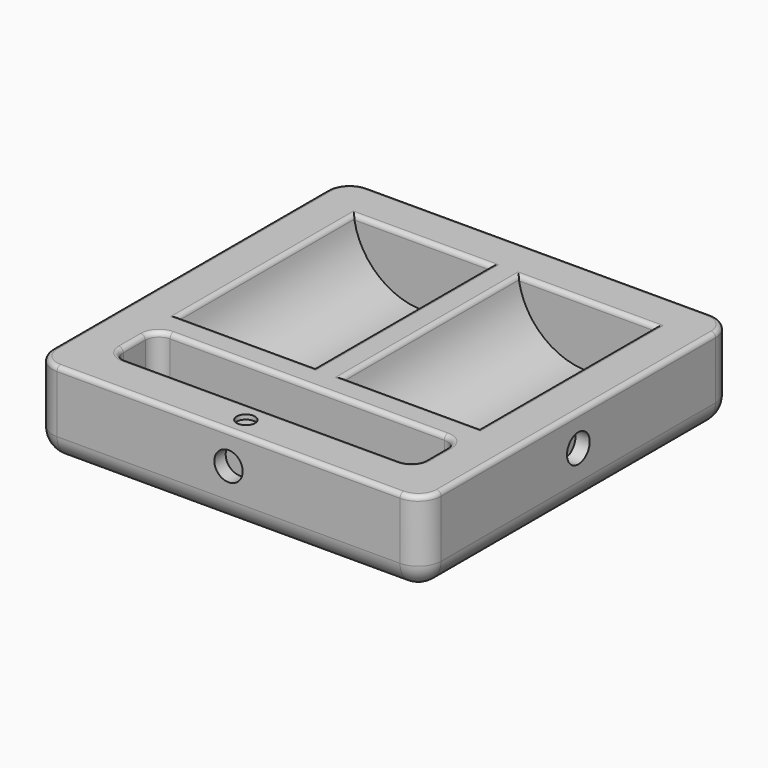
from build123d import *

# Parameters (mm, degrees)
F0_W      = 85
F0_H      = 85
F0_R      = 2
F3_DEPTH  = 18.5
F4_DEPTH  = 14
F5_R      = 5
F6_R      = 3
F7_R      = 3.1
F8_DEPTH  = 3.1
F9_R      = 3.1
F10_DEPTH = 3.1
F11_R     = 3.1
F12_DEPTH = 3.1
F13_R     = 3.1
F14_DEPTH = 3.1
F15_DEPTH = 1
F18_DEPTH = 48
F19_R     = 1
F20_ANGLE = 180


# Not quite as in the source:
# - a feature names something its author has since deleted; it is built from what else it names


with BuildPart() as f3:
    # F0 (on Top) → F3 (new body)
    with BuildSketch(Plane.XY):
        Rectangle(F0_W, F0_H)
        with BuildLine():
            ThreePointArc((-33, 30), (-32.1213203436, 32.1213203436), (-30, 33))
            Line((-30, 33), (30, 33))
            ThreePointArc((30, 33), (32.1213203436, 32.1213203436), (33, 30))
            Line((33, 30), (33, 24))
            ThreePointArc((33, 24), (32.1213203436, 21.8786796564), (30, 21))
            Line((30, 21), (-30, 21))
            ThreePointArc((-30, 21), (-32.1213203436, 21.8786796564), (-33, 24))
            Line((-33, 24), (-33, 30))
        make_face(mode=Mode.SUBTRACT)
        with Locations((0, 37.75)):
            Circle(F0_R, mode=Mode.SUBTRACT)
        with BuildLine():
            Line((30, 33), (-30, 33))
            ThreePointArc((-30, 33), (-32.1213203436, 32.1213203436), (-33, 30))
            Line((-33, 30), (-33, 24))
            ThreePointArc((-33, 24), (-32.1213203436, 21.8786796564), (-30, 21))
            Line((-30, 21), (30, 21))
            ThreePointArc((30, 21), (32.1213203436, 21.8786796564), (33, 24))
            Line((33, 24), (33, 30))
            ThreePointArc((33, 30), (32.1213203436, 32.1213203436), (30, 33))
        make_face()
        with Locations((0, 37.75)):
            Circle(F0_R)
    extrude(amount=F3_DEPTH)

    # F0 (on Top) → F4 (cut)
    with BuildSketch(Plane.XY):
        with BuildLine():
            Line((30, 33), (-30, 33))
            ThreePointArc((-30, 33), (-32.1213203436, 32.1213203436), (-33, 30))
            Line((-33, 30), (-33, 24))
            ThreePointArc((-33, 24), (-32.1213203436, 21.8786796564), (-30, 21))
            Line((-30, 21), (30, 21))
            ThreePointArc((30, 21), (32.1213203436, 21.8786796564), (33, 24))
            Line((33, 24), (33, 30))
            ThreePointArc((33, 30), (32.1213203436, 32.1213203436), (30, 33))
        make_face()
    extrude(amount=F4_DEPTH, mode=Mode.SUBTRACT)

    # F5
    f5_edges = [f3.edges().sort_by_distance(p)[0] for p in [
        (0, 42.5, 18.5),
        (-42.5, 0, 18.5),
        (0, -42.5, 18.5),
        (42.5, 0, 18.5),
        (42.5, 42.5, 9.25),
        (-42.5, 42.5, 9.25),
        (-42.5, -42.5, 9.25),
        (42.5, -42.5, 9.25),
    ]]
    fillet(f5_edges, radius=F5_R)

    # F6
    f6_edges = [f3.edges().sort_by_distance(p)[0] for p in [
        (0, 33, 14),
        (-32.12132, 32.12132, 14),
        (-33, 27, 14),
        (-32.12132, 21.87868, 14),
        (0, 21, 14),
        (32.12132, 21.87868, 14),
        (33, 27, 14),
        (32.12132, 32.12132, 14),
    ]]
    fillet(f6_edges, radius=F6_R)

    # F7 (on face) → F8 (cut)
    with BuildSketch(Plane.XZ.offset(42.5)):
        with Locations((0, 7)):
            Circle(F7_R)
    extrude(amount=-F8_DEPTH, mode=Mode.SUBTRACT)

    # F9 (on face) → F10 (cut)
    with BuildSketch(Plane(origin=(0, 42.5, 0), x_dir=(-1, 0, 0), z_dir=(0, 1, 0))):
        with Locations((0, 7)):
            Circle(F9_R)
    extrude(amount=-F10_DEPTH, mode=Mode.SUBTRACT)

    # F11 (on face) → F12 (cut)
    with BuildSketch(Plane(origin=(-42.5, 0, 0), x_dir=(0, -1, 0), z_dir=(-1, 0, 0))):
        with Locations((0, 7)):
            Circle(F11_R)
    extrude(amount=-F12_DEPTH, mode=Mode.SUBTRACT)

    # F13 (on face) → F14 (cut)
    with BuildSketch(Plane.YZ.offset(42.5)):
        with Locations((0, 7)):
            Circle(F13_R)
    extrude(amount=-F14_DEPTH, mode=Mode.SUBTRACT)

    # F0 (on Top) → F15 (cut)
    with BuildSketch(Plane.XY):
        with Locations((0, 37.75)):
            Circle(F0_R)
    extrude(amount=F15_DEPTH, mode=Mode.SUBTRACT)

    # F17 (on offset) → F18 (cut)
    with BuildSketch(Plane(origin=(0, 15, 0), x_dir=(-1, 0, 0), z_dir=(0, 1, 0))):
        with BuildLine():
            Line((-33, 0), (-3, 0))
            ThreePointArc((-3, 0), (-18, 13.5), (-33, 0))
        make_face()
        with BuildLine():
            Line((3, 0), (33, 0))
            ThreePointArc((33, 0), (18, 13.5), (3, 0))
        make_face()
    extrude(amount=-F18_DEPTH, mode=Mode.SUBTRACT)

    # F19
    f19_edges = [f3.edges().sort_by_distance(p)[0] for p in [
        (-42.5, 0, 0),
        (-33, -9, 0),
        (-18, 15, 0),
        (-3, -9, 0),
        (-18, -33, 0),
        (3, -9, 0),
        (18, -33, 0),
        (33, -9, 0),
        (18, 15, 0),
        (0, 21, 0),
    ]]
    fillet(f19_edges, radius=F19_R)


with BuildPart() as f3_1:
    # F20: moved
    add(f3.part.rotate(Axis((0, 0, 0), (1, 0, 0)), F20_ANGLE))


solid = f3_1.part
